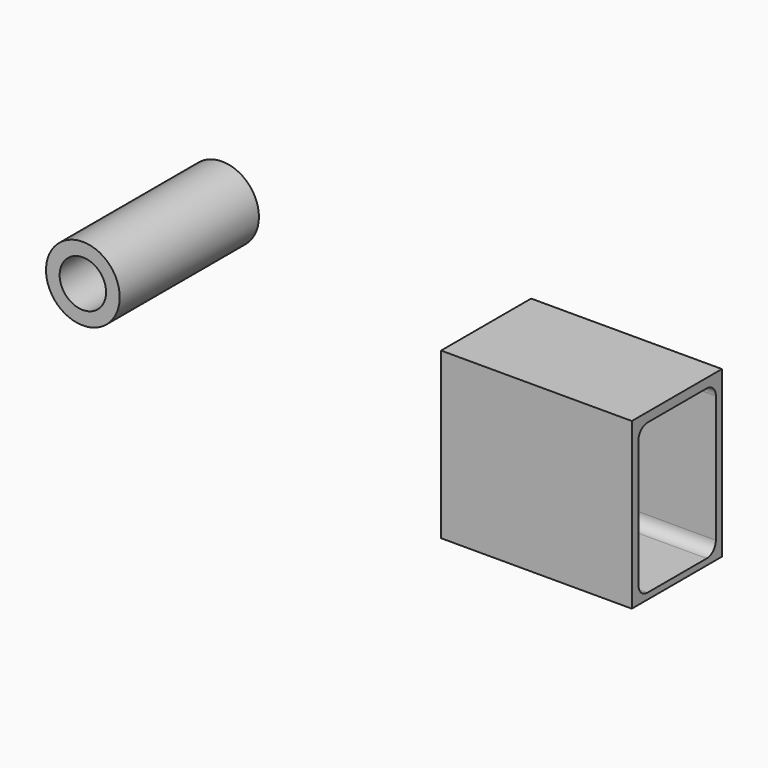
from build123d import *

# Parameters (mm, degrees)
F0_R     = 16.4582820338
F0_R_2   = 10.3759
F1_DEPTH = 77.724
F2_R     = 10.3759
F3_DEPTH = 121.158
F4_W     = 85.2083563805
F4_H     = 73.7946406007
F5_DEPTH = 50.292
F6_W     = 43.2375106029
F6_H     = 66.885214299
F7_DEPTH = 214.122
F8_R     = 5.08


with BuildPart() as f1:
    # F0 (on Front) → F1 (new body)
    with BuildSketch(Plane.XZ):
        with Locations((-66.5547922254, 27.202360332)):
            Circle(F0_R)
        with Locations((-66.5547922254, 27.202360332)):
            Circle(F0_R_2, mode=Mode.SUBTRACT)
        with Locations((-66.5547922254, 27.202360332)):
            Circle(F0_R_2)
    extrude(amount=F1_DEPTH)

    # F2 (on face) → F3 (cut)
    with BuildSketch(Plane(origin=(0, 0, 0), x_dir=(-1, 0, 0), z_dir=(0, 1, 0))):
        with Locations((66.5547922254, 27.202360332)):
            Circle(F2_R)
    extrude(amount=-F3_DEPTH, mode=Mode.SUBTRACT)


with BuildPart() as f5:
    # F4 (on Front) → F5 (new body)
    with BuildSketch(Plane.XZ):
        with Locations((114.0915453434, -2.257052809)):
            Rectangle(F4_W, F4_H)
    extrude(amount=F5_DEPTH)

    # F6 (on face) → F7 (cut)
    with BuildSketch(Plane.YZ.offset(156.6957235336)):
        with Locations((-25.0060728285, -2.9566902667)):
            Rectangle(F6_W, F6_H)
    extrude(amount=-F7_DEPTH, mode=Mode.SUBTRACT)

    # F8
    f8_edges = [f5.edges().sort_by_distance(p)[0] for p in [
        (114.091545, -3.387318, 30.485917),
        (114.091545, -46.624828, 30.485917),
        (114.091545, -46.624828, -36.399297),
        (114.091545, -3.387318, -36.399297),
    ]]
    fillet(f8_edges, radius=F8_R)


solid = Compound([f1.part, f5.part])
